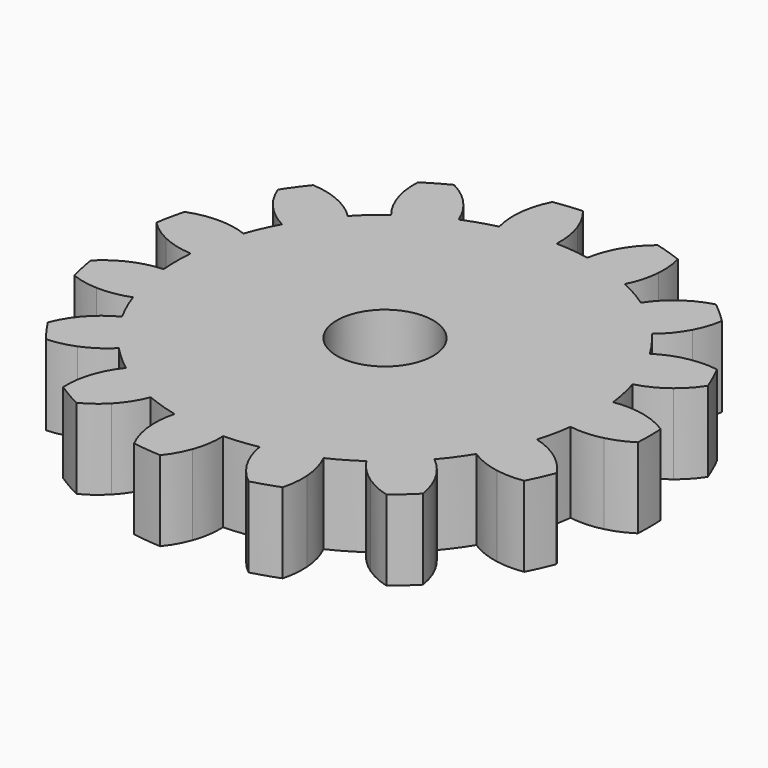
from build123d import *

# Parameters (mm, degrees)
F0_R            = 3
F1_DEPTH        = 5
F1_COPIES_COUNT = 15


# Not quite as in the source:
# - a feature of the source that left no trace in its solid (it failed there, or was rolled back) is left out
# - a pattern or mirror of a feature is missing from the dataset's text; its kind, count and spacing are read off the source's solid


with BuildPart() as f1:
    # F0 (on Top) → F1 (new body)
    with BuildSketch(Plane.XY):
        with BuildLine():
            ThreePointArc((-2.9988420109, 12.6493852259), (-8.0627245351, -10.1976699824), (13, 0))
            ThreePointArc((13, 0), (9.2990218739, 9.0845028587), (0.3033550478, 12.9964601225))
            ThreePointArc((0.3033550478, 12.9964601225), (-1.3588700225, 12.9287846398), (-2.9988420109, 12.6493852259))
        make_face()
        Circle(F0_R, mode=Mode.SUBTRACT)
        with BuildLine():
            ThreePointArc((-2.9988420109, 12.6493852259), (-1.3588700225, 12.9287846398), (0.3033550478, 12.9964601225))
            ThreePointArc((0.3033550478, 12.9964601225), (0.2516824721, 14.0133717643), (0, 15))
            ThreePointArc((0, 15), (-0.3567287211, 15.774579327), (-0.837788828, 16.478716876))
            ThreePointArc((-0.837788828, 16.478716876), (-1.7247092492, 16.409512374), (-2.6066367562, 16.2928034672))
            ThreePointArc((-2.6066367562, 16.2928034672), (-2.9307861171, 15.5040349929), (-3.1186753623, 14.672214011))
            ThreePointArc((-3.1186753623, 14.672214011), (-3.1597264238, 13.6548182411), (-2.9988420109, 12.6493852259))
        make_face()
    extrude(amount=F1_DEPTH)

    # F1_copies: F1 ×15 about axis
    f1_copies_axis = Axis((0, 0, 0), (0, 0, 1))


with BuildPart() as f1_1:
    add(f1.part)
    for i in range(1, F1_COPIES_COUNT):
        add(f1.part.rotate(f1_copies_axis, i * 360 / F1_COPIES_COUNT))


solid = f1_1.part
